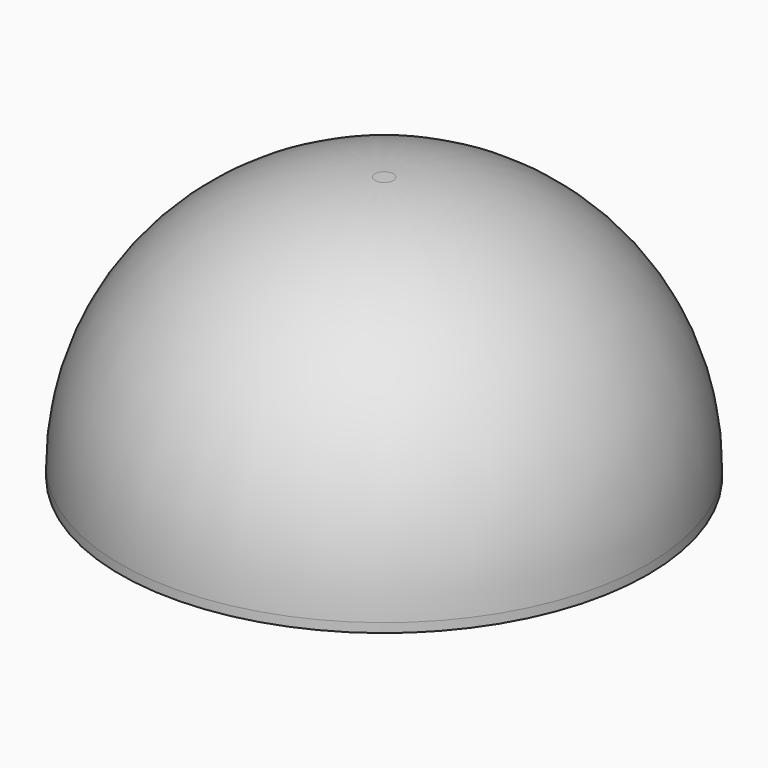
from build123d import *

# Parameters (mm, degrees)
F0_R     = 50
F1_DEPTH = 50
F2_R     = 48.26
F3_T     = -2.54


with BuildPart() as f1:
    # F0 (on Top) → F1 (new body)
    with BuildSketch(Plane.XY):
        Circle(F0_R)
    extrude(amount=F1_DEPTH)

    # F2
    f2_edges = [f1.edges().sort_by_distance(p)[0] for p in [
        (-50, 0, 50),
    ]]
    fillet(f2_edges, radius=F2_R)

    # F3
    f3_openings = [f1.faces().sort_by_distance(p)[0] for p in [
        (0, 0, 0),
    ]]
    offset(amount=F3_T, openings=f3_openings)


solid = f1.part
